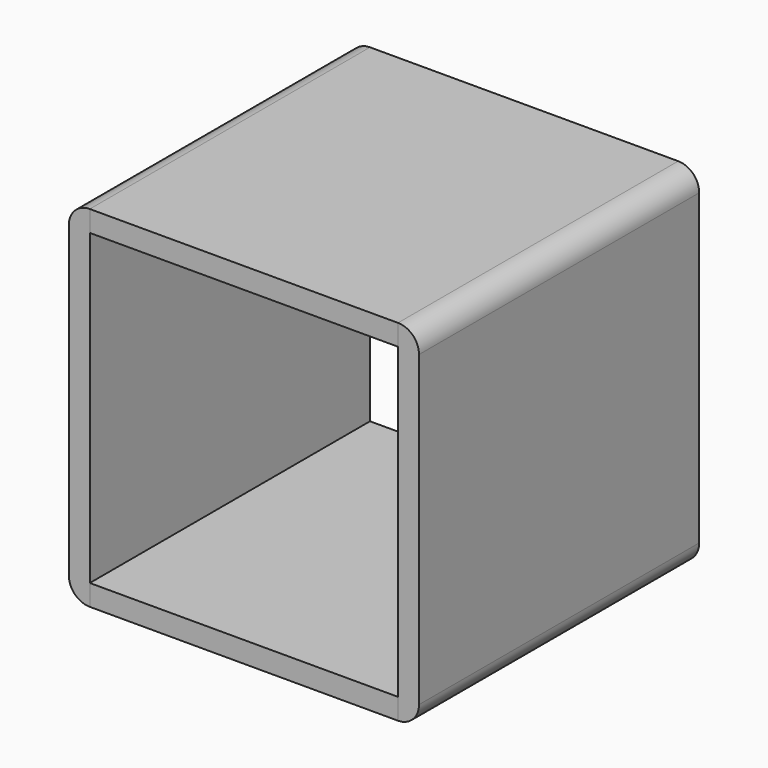
from build123d import *

# Parameters (mm, degrees)
F2_DEPTH = 200
F1_W     = 176
F1_H     = 12
F3_DEPTH = 200
F4_R     = 11.99999
F4_2_R   = 11.99999


# Not quite as in the source:
# - a fillet or chamfer is up to 0.001 mm smaller than in the source, because OpenCascade refuses the exact size


with BuildPart() as f2:
    # F1 (on Front) → F2 (new body)
    with BuildSketch(Plane.XZ):
        Polygon((-37.4641348869, 97.1549547033), (-49.4641348869, 97.1549547033), (-49.4641348869, -102.8450452967), (-37.4641348869, -102.8450452967), (-37.4641348869, -90.8450452967), (-37.4641348869, 85.1549547033), align=None)
    extrude(amount=F2_DEPTH)

    # F4#2 (radius 12 in the source; OpenCascade refuses exactly that, so slightly less here)
    f4_2_edges = [f2.edges().sort_by_distance(p)[0] for p in [
        (-49.464135, -100, -102.845045),
        (-49.464135, -100, 97.154955),
    ]]
    fillet(f4_2_edges, radius=F4_2_R)


with BuildPart() as f2b:
    # F1 (on Front) → F2, piece 2 (new body)
    with BuildSketch(Plane.XZ):
        Polygon((150.5358651131, 97.1549547033), (138.5358651131, 97.1549547033), (138.5358651131, 85.1549547033), (138.5358651131, -90.8450452967), (138.5358651131, -102.8450452967), (150.5358651131, -102.8450452967), align=None)
    extrude(amount=F2_DEPTH)

    # F4 (radius 12 in the source; OpenCascade refuses exactly that, so slightly less here)
    f4_edges = [f2b.edges().sort_by_distance(p)[0] for p in [
        (150.535865, -100, -102.845045),
        (150.535865, -100, 97.154955),
    ]]
    fillet(f4_edges, radius=F4_R)


with BuildPart() as f3:
    # F1 (on Front) → F3 (new body)
    with BuildSketch(Plane.XZ):
        with Locations((50.5358651131, 91.1549547033)):
            Rectangle(F1_W, F1_H)
    extrude(amount=F3_DEPTH)


with BuildPart() as f3b:
    # F1 (on Front) → F3, piece 2 (new body)
    with BuildSketch(Plane.XZ):
        with Locations((50.5358651131, -96.8450452967)):
            Rectangle(F1_W, F1_H)
    extrude(amount=F3_DEPTH)


solid = Compound([f2.part, f2b.part, f3.part, f3b.part])
